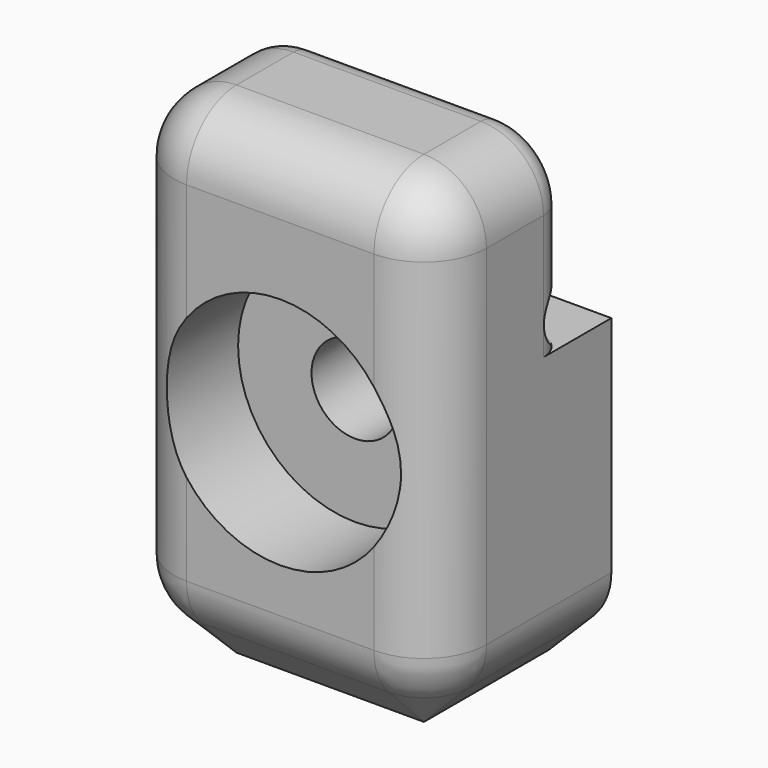
from build123d import *

# Parameters (mm, degrees)
F1_DEPTH     = 25.4
F2_R         = 3.556
F3_DEPTH     = 17.78
F4_R         = 9.525
F4_R_2       = 3.556
F5_DEPTH     = 7.62
F6_T1_DEPTH  = 48.26
F6_T3_DEPTH  = 20.828
F6_T5_DEPTH  = 15.24
F6_S9_W      = 5.08
F6_S9_H      = 5.08
F6_T10_DEPTH = 5.08
F6_S15_W     = 5.08
F6_S15_H     = 5.08
F6_T16_DEPTH = 5.08
F7_SIZE      = 5.07999
F8_R         = 5.08
F9_T3_DEPTH  = 15.24
F9_T6_DEPTH  = 11.413497326
F9_T10_DEPTH = 11.413497326
F9_T14_ANGLE = 89.9999999979
F9_T17_ANGLE = 89.9999999979


# Not quite as in the source:
# - a fillet or chamfer that OpenCascade refuses, or shapes differently, is made with other operations: its cross-section is extruded or revolved along the edge and cut away or added
# - a fillet or chamfer is up to 0.001 mm smaller than in the source, because OpenCascade refuses the exact size


with BuildPart() as f1:
    # F0 (on Right) → F1 (new body)
    with BuildSketch(Plane.YZ):
        with BuildLine():
            Line((0, -25.4), (0, 0))
            Line((0, 0), (-4.572, 0))
            ThreePointArc((-4.572, 0), (-6.858, 2.286), (-4.572, 4.572))
            Line((-4.572, 4.572), (-4.572, 15.24))
            Line((-4.572, 15.24), (-17.78, 15.24))
            Line((-17.78, 15.24), (-17.78, 0))
            Line((-17.78, 0), (-17.78, -25.4))
            Line((-17.78, -25.4), (0, -25.4))
        make_face()
    extrude(amount=F1_DEPTH)

    # F2 (on face) → F3 (cut, through all)
    with BuildSketch(Plane(origin=(0, 0, 0), x_dir=(-1, 0, 0), z_dir=(0, 1, 0))):
        with Locations((-12.7, -5.08)):
            Circle(F2_R)
    extrude(amount=-F3_DEPTH, mode=Mode.SUBTRACT)

    # F4 (on face) → F5 (cut)
    with BuildSketch(Plane.XZ.offset(17.78)):
        with Locations((12.7, -5.08)):
            Circle(F4_R)
        with Locations((12.7, -5.08)):
            Circle(F4_R_2, mode=Mode.SUBTRACT)
    extrude(amount=-F5_DEPTH, mode=Mode.SUBTRACT)

    # F6: fillet of radius 5.08 on 5 edges, made by hand

    # F6_s2 → F6_t1 (cut)
    with BuildSketch(Plane.XY.offset(-38.1)):
        with BuildLine():
            ThreePointArc((5.08, -17.78), (1.4878975516, -16.2921024484), (0, -12.7))
            Line((0, -12.7), (0, -17.78))
            Line((0, -17.78), (5.08, -17.78))
        make_face()
        with BuildLine():
            ThreePointArc((20.32, -17.78), (23.9121024484, -16.2921024484), (25.4, -12.7))
            Line((25.4, -12.7), (25.4, -17.78))
            Line((25.4, -17.78), (20.32, -17.78))
        make_face()
    extrude(amount=F6_T1_DEPTH, mode=Mode.SUBTRACT)

    # F6_s4 → F6_t3 (cut)
    with BuildSketch(Plane.XZ.offset(-8.128)):
        with BuildLine():
            ThreePointArc((20.32, 15.24), (23.9121024484, 13.7521024484), (25.4, 10.16))
            Line((25.4, 10.16), (25.4, 15.24))
            Line((25.4, 15.24), (20.32, 15.24))
        make_face()
        with BuildLine():
            ThreePointArc((5.08, 15.24), (1.4878975516, 13.7521024484), (0, 10.16))
            Line((0, 10.16), (0, 15.24))
            Line((0, 15.24), (5.08, 15.24))
        make_face()
    extrude(amount=F6_T3_DEPTH, mode=Mode.SUBTRACT)

    # F6_s6 → F6_t5 (cut)
    with BuildSketch(Plane.YZ.offset(5.08)):
        with BuildLine():
            ThreePointArc((-17.78, 10.16), (-16.2921024484, 13.7521024484), (-12.7, 15.24))
            Line((-12.7, 15.24), (-17.78, 15.24))
            Line((-17.78, 15.24), (-17.78, 10.16))
        make_face()
    extrude(amount=F6_T5_DEPTH, mode=Mode.SUBTRACT)


with BuildPart() as f6_tool8:
    # F6_s9 → F6_t10 (new body)
    with BuildSketch(Plane.YZ.offset(5.08)):
        with Locations((-15.24, 12.7)):
            Rectangle(F6_S9_W, F6_S9_H)
    extrude(amount=-F6_T10_DEPTH)

    # F6_s11 → F6_t12 (revolve, cut)
    with BuildSketch(Plane(origin=(5.08, -12.7, 10.16), x_dir=(0, 0.7071067812, -0.7071067812), z_dir=(0, 0.7071067812, 0.7071067812))):
        with BuildLine():
            ThreePointArc((0, -5.08), (5.08, 0), (0, 5.08))
            Line((0, 5.08), (0, -5.08))
        make_face()
    revolve(axis=Axis((5.08, -12.7, 10.16), (-1, 0, 0)), mode=Mode.SUBTRACT)


with BuildPart() as f1_1:
    add(f1.part)

    # F6_t7: cut F6_tool8
    add(f6_tool8.part, mode=Mode.SUBTRACT)


with BuildPart() as f6_tool14:
    # F6_s15 → F6_t16 (new body)
    with BuildSketch(Plane.YZ.offset(20.32)):
        with Locations((-15.24, 12.7)):
            Rectangle(F6_S15_W, F6_S15_H)
    extrude(amount=F6_T16_DEPTH)

    # F6_s17 → F6_t18 (revolve, cut)
    with BuildSketch(Plane(origin=(20.32, -12.7, 10.16), x_dir=(0, 0.7071067812, -0.7071067812), z_dir=(0, -0.7071067812, -0.7071067812))):
        with BuildLine():
            ThreePointArc((0, -5.08), (5.08, 0), (0, 5.08))
            Line((0, 5.08), (0, -5.08))
        make_face()
    revolve(axis=Axis((20.32, -12.7, 10.16), (1, 0, 0)), mode=Mode.SUBTRACT)


with BuildPart() as f1_2:
    add(f1_1.part)

    # F6_t13: cut F6_tool14
    add(f6_tool14.part, mode=Mode.SUBTRACT)

    # F7 (size 5.08 in the source; OpenCascade refuses exactly that, so slightly less here)
    f7_edges = [f1_2.edges().sort_by_distance(p)[0] for p in [
        (12.7, -17.78, -25.4),
    ]]
    chamfer(f7_edges, length=F7_SIZE)

    # F8
    f8_edges = [f1_2.edges().sort_by_distance(p)[0] for p in [
        (12.7, -17.78, -20.32001),
        (0, -6.35, -20.32001),
        (25.4, -6.35, -20.32001),
        (1.487898, -16.292102, -20.32001),
        (23.912102, -16.292102, -20.32001),
    ]]
    fillet(f8_edges, radius=F8_R)

    # F9: fillet of radius 2.3301989304 on 5 edges, made by hand


with BuildPart() as f9_tool1:
    # F9_s2 → F9_t3 (new body)
    with BuildSketch(Plane.YZ.offset(5.08)):
        with BuildLine():
            ThreePointArc((-4.572, 12.9098010696), (-5.2544994652, 14.5575005348), (-6.9021989304, 15.24))
            Line((-6.9021989304, 15.24), (-4.572, 15.24))
            Line((-4.572, 15.24), (-4.572, 12.9098010696))
        make_face()
    extrude(amount=F9_T3_DEPTH)


with BuildPart() as f9_tool4:
    # F9_s5 → F9_t6 (new body)
    with BuildSketch(Plane.XY.offset(-1.253497326)):
        with BuildLine():
            ThreePointArc((0, -6.9021989304), (0.6824994652, -5.2544994652), (2.3301989304, -4.572))
            Line((2.3301989304, -4.572), (0, -4.572))
            Line((0, -4.572), (0, -6.9021989304))
        make_face()
    extrude(amount=F9_T6_DEPTH)

    split(bisect_by=Plane.XY, keep=Keep.TOP)


with BuildPart() as f9_tool8:
    # F9_s9 → F9_t10 (new body)
    with BuildSketch(Plane.XY.offset(-1.253497326)):
        with BuildLine():
            ThreePointArc((25.4, -6.9021989304), (24.7175005348, -5.2544994652), (23.0698010696, -4.572))
            Line((23.0698010696, -4.572), (25.4, -4.572))
            Line((25.4, -4.572), (25.4, -6.9021989304))
        make_face()
    extrude(amount=F9_T10_DEPTH)

    split(bisect_by=Plane.XY, keep=Keep.TOP)


with BuildPart() as f9_tool12:
    # F9_s13 → F9_t14 (revolve)
    with BuildSketch(Plane.XY.offset(10.1599999999)):
        with BuildLine():
            ThreePointArc((0, -6.9021989304), (0.6824994652, -5.2544994652), (2.3301989304, -4.572))
            Line((2.3301989304, -4.572), (0, -4.572))
            Line((0, -4.572), (0, -6.9021989304))
        make_face()
    revolve(axis=Axis((5.0800000001, -4.572, 10.1599999999), (0, 1, 0)), revolution_arc=F9_T14_ANGLE)


with BuildPart() as f9_tool15:
    # F9_s16 → F9_t17 (revolve)
    with BuildSketch(Plane.YZ.offset(20.3199999999)):
        with BuildLine():
            ThreePointArc((-4.572, 12.9098010696), (-5.2544994652, 14.5575005348), (-6.9021989304, 15.24))
            Line((-6.9021989304, 15.24), (-4.572, 15.24))
            Line((-4.572, 15.24), (-4.572, 12.9098010696))
        make_face()
    revolve(axis=Axis((20.3199999999, -4.572, 10.1599999999), (0, 1, 0)), revolution_arc=F9_T17_ANGLE)


with BuildPart() as f1_3:
    add(f1_2.part)

    # F9_t18: cut F9_tool1, F9_tool4, F9_tool8, F9_tool12, F9_tool15
    add([f9_tool1.part, f9_tool4.part, f9_tool8.part, f9_tool12.part, f9_tool15.part], mode=Mode.SUBTRACT)


solid = f1_3.part
